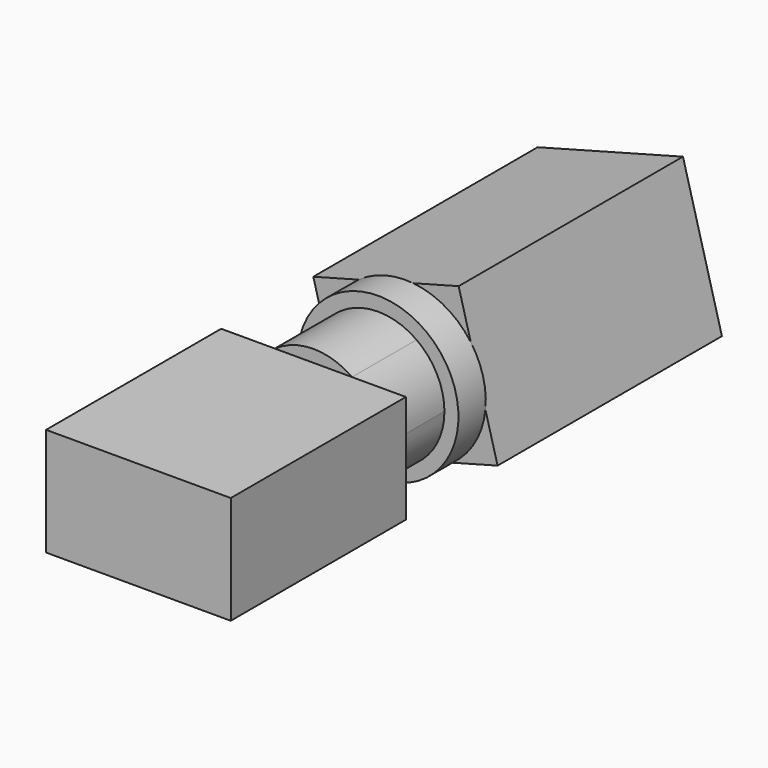
from build123d import *

# Parameters (mm, degrees)
F1_DEPTH = 5.9
F2_DEPTH = 16
F3_R     = 5.875
F3_R_2   = 4.85
F4_DEPTH = 2.5
F6_DEPTH = 20.5


with BuildPart() as f1:
    # F0 (on Front) → F1 (new body)
    with BuildSketch(Plane.XZ):
        with BuildLine():
            Line((-2.8142494559, -3.95), (2.8142494559, -3.95))
            ThreePointArc((2.8142494559, -3.95), (4.311125715, -2.2218674734), (4.85, 0))
            ThreePointArc((4.85, 0), (4.311125715, 2.2218674734), (2.8142494559, 3.95))
            Line((2.8142494559, 3.95), (-2.8142494559, 3.95))
            ThreePointArc((-2.8142494559, 3.95), (-4.85, 0), (-2.8142494559, -3.95))
        make_face()
        with BuildLine():
            ThreePointArc((-2.8142494559, -3.95), (0, -4.85), (2.8142494559, -3.95))
            Line((2.8142494559, -3.95), (-2.8142494559, -3.95))
        make_face()
        with BuildLine():
            Line((-2.8142494559, 3.95), (2.8142494559, 3.95))
            ThreePointArc((2.8142494559, 3.95), (0, 4.85), (-2.8142494559, 3.95))
        make_face()
    extrude(amount=-F1_DEPTH)

    # F0 (on Front) → F2 (join)
    with BuildSketch(Plane.XZ):
        with BuildLine():
            Line((-6.75, -3.95), (-2.8142494559, -3.95))
            ThreePointArc((-2.8142494559, -3.95), (-4.85, 0), (-2.8142494559, 3.95))
            Line((-2.8142494559, 3.95), (-6.75, 3.95))
            Line((-6.75, 3.95), (-6.75, -3.95))
        make_face()
        with BuildLine():
            Line((-2.8142494559, -3.95), (2.8142494559, -3.95))
            ThreePointArc((2.8142494559, -3.95), (4.311125715, -2.2218674734), (4.85, 0))
            ThreePointArc((4.85, 0), (4.311125715, 2.2218674734), (2.8142494559, 3.95))
            Line((2.8142494559, 3.95), (-2.8142494559, 3.95))
            ThreePointArc((-2.8142494559, 3.95), (-4.85, 0), (-2.8142494559, -3.95))
        make_face()
        with BuildLine():
            Line((2.8142494559, -3.95), (6.75, -3.95))
            Line((6.75, -3.95), (6.75, 3.95))
            Line((6.75, 3.95), (2.8142494559, 3.95))
            ThreePointArc((2.8142494559, 3.95), (4.311125715, 2.2218674734), (4.85, 0))
            ThreePointArc((4.85, 0), (4.311125715, -2.2218674734), (2.8142494559, -3.95))
        make_face()
    extrude(amount=F2_DEPTH)

    # F3 (on face) → F4 (join)
    with BuildSketch(Plane(origin=(0, 5.9, 0), x_dir=(-1, 0, 0), z_dir=(0, 1, 0))):
        Circle(F3_R)
        Circle(F3_R_2, mode=Mode.SUBTRACT)
        Circle(F3_R_2)
    extrude(amount=F4_DEPTH)

    # F5 (on face) → F6 (join)
    with BuildSketch(Plane(origin=(0, 8.4, 0), x_dir=(-1, 0, 0), z_dir=(0, 1, 0))):
        Polygon((-6.7360967927, -3.8890872965), (3.8890872965, -6.7360967927), (6.7360967927, 3.8890872965), (-3.8890872965, 6.7360967927), align=None)
    extrude(amount=F6_DEPTH)


solid = f1.part
